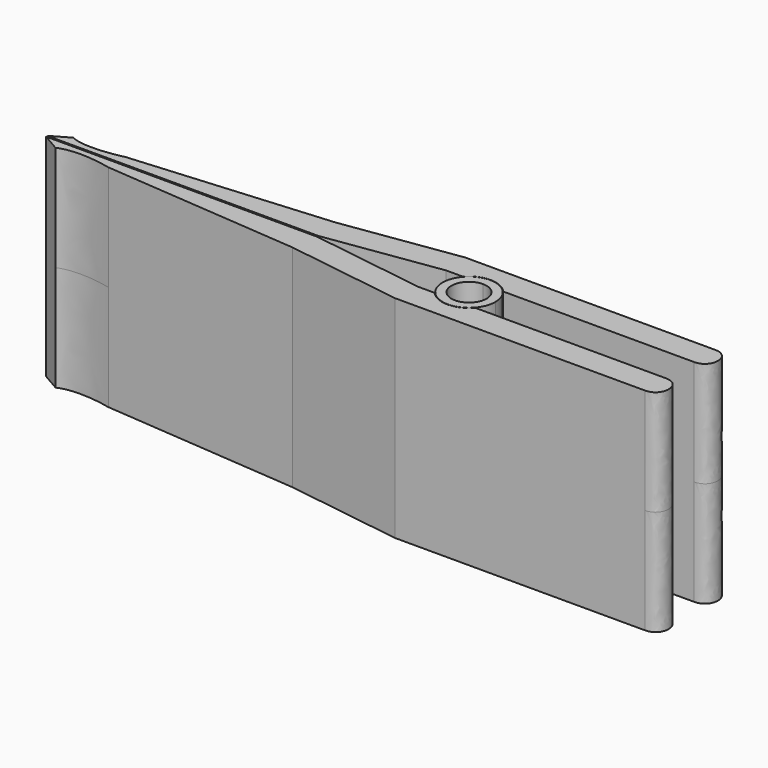
from build123d import *

# Parameters (mm, degrees)
F1_DEPTH = 9.525
F2_DEPTH = 6.35
F5_DEPTH = 3.175
F9_DEPTH = 3.175


# Not quite as in the source:
# - a feature of the source that left no trace in its solid (it failed there, or was rolled back) is left out


with BuildPart() as f1:
    # F0 (on Top) → F1 (new body, symmetric)
    with BuildSketch(Plane.XY):
        with BuildLine():
            Line((19.0503296435, -3.175), (1.8172541787, -3.175))
            ThreePointArc((1.8172541787, -3.175), (0, -4.0005), (-1.8172541787, -3.175))
            Line((-1.8172541787, -3.175), (-3.3368981663, -3.175))
            Line((-3.3368981663, -3.175), (-13.6596335379, -1.6637))
            Line((-13.6596335379, -1.6637), (-38.1, -1.6637))
            Line((-38.1, -1.6637), (-36.5125, -2.5802435523))
            add(Edge.make_bspline(
                [(-36.5125, -2.5802435523), (-35.5840288103, -2.1219717762), (-33.6853526533, -2.1219717762), (-31.75, -2.5802435523)],
                knots=[0, 0, 0, 0, 4.7625, 4.7625, 4.7625, 4.7625], degree=3))
            Line((-31.75, -2.5802435523), (-13.9957684352, -4.0211232241))
            Line((-13.9957684352, -4.0211232241), (-3.5102874127, -5.55625))
            Line((-3.5102874127, -5.55625), (19.0503296435, -5.55625))
            add(Edge.make_bspline(
                [(19.0503296435, -5.55625), (20.6378296435, -5.55625), (20.6378296435, -3.175), (19.0503296435, -3.175)],
                knots=[0, 0, 0, 0, 2.38125, 2.38125, 2.38125, 2.38125], degree=3))
        make_face()
    extrude(amount=F1_DEPTH, both=True)


with BuildPart() as f1b:
    # F0 (on Top) → F1, piece 2 (new body, symmetric)
    with BuildSketch(Plane.XY):
        with BuildLine():
            Line((1.8172541787, 0), (19.05, 0))
            add(Edge.make_bspline(
                [(19.05, 2.38125), (20.6375, 2.38125), (20.6375, 0), (19.05, 0)],
                knots=[0, 0, 0, 0, 2.38125, 2.38125, 2.38125, 2.38125], degree=3))
            Line((19.05, 2.38125), (-3.5102874127, 2.38125))
            Line((-3.5102874127, 2.38125), (-13.9957684352, 0.8461232241))
            Line((-13.9957684352, 0.8461232241), (-31.75, -0.5947564477))
            add(Edge.make_bspline(
                [(-36.5125, -0.5947564477), (-35.5840288103, -1.0530282238), (-33.6853526533, -1.0530282238), (-31.75, -0.5947564477)],
                knots=[0, 0, 0, 0, 4.7625, 4.7625, 4.7625, 4.7625], degree=3))
            Line((-36.5125, -0.5947564477), (-38.1, -1.5113))
            Line((-38.1, -1.5113), (-13.6596335379, -1.5113))
            Line((-13.6596335379, -1.5113), (-3.3368981663, 0))
            Line((-3.3368981663, 0), (-1.8172541787, 0))
            ThreePointArc((-1.8172541787, 0), (0, 0.8255), (1.8172541787, 0))
        make_face()
    extrude(amount=F1_DEPTH, both=True)

    # F0 (on Top) → F2 (join, symmetric)
    with BuildSketch(Plane.XY):
        with BuildLine():
            Line((0, 0), (1.7748789571, 0))
            ThreePointArc((1.7748789571, 0), (0, 0.79375), (-1.7748789571, 0))
            Line((-1.7748789571, 0), (0, 0))
        make_face()
        with BuildLine():
            Line((1.7748789571, 0), (1.8172541787, 0))
            ThreePointArc((1.8172541787, 0), (0, 0.8255), (-1.8172541787, 0))
            Line((-1.8172541787, 0), (-1.7748789571, 0))
            ThreePointArc((-1.7748789571, 0), (0, 0.79375), (1.7748789571, 0))
        make_face()
    extrude(amount=F2_DEPTH, both=True)

    # F3: union 

    # F4 (on face) → F5 (join)
    with BuildSketch(Plane.XY.offset(6.35)):
        with BuildLine():
            ThreePointArc((-1.7748789571, 0), (-0.8496826013, -3.8119979298), (2.38125, -1.5875))
            ThreePointArc((2.38125, -1.5875), (2.2244979298, -0.7378173987), (1.7748789571, 0))
            Line((1.7748789571, 0), (0, 0))
            Line((0, 0), (-1.7748789571, 0))
        make_face()
        with BuildLine():
            ThreePointArc((1.5875, -1.5875), (-1.1225320151, -2.7100320151), (0, 0))
            ThreePointArc((0, 0), (1.1225320151, -0.4649679849), (1.5875, -1.5875))
        make_face(mode=Mode.SUBTRACT)
        with BuildLine():
            Line((0, 0), (1.7748789571, 0))
            ThreePointArc((1.7748789571, 0), (0, 0.79375), (-1.7748789571, 0))
            Line((-1.7748789571, 0), (0, 0))
        make_face()
    extrude(amount=F5_DEPTH)

    # F8 (on face) → F9 (join)
    with BuildSketch(Plane(origin=(0, 0, -6.35), x_dir=(1, 0, 0), z_dir=(0, 0, -1))):
        with BuildLine():
            Line((-3e-10, 0), (-1.7748789571, 0))
            ThreePointArc((-1.7748789571, 0), (0, -0.79375), (1.7748789571, 0))
            Line((1.7748789571, 0), (-3e-10, 0))
        make_face()
        with BuildLine():
            ThreePointArc((1.7748789571, 0), (0, -0.79375), (-1.7748789571, 0))
            Line((-1.7748789571, 0), (-1.8172541787, 0))
            ThreePointArc((-1.8172541787, 0), (0, -0.8255), (1.8172541787, 0))
            Line((1.8172541787, 0), (1.7748789571, 0))
        make_face()
    extrude(amount=F9_DEPTH)


solid = Compound([f1.part, f1b.part])
